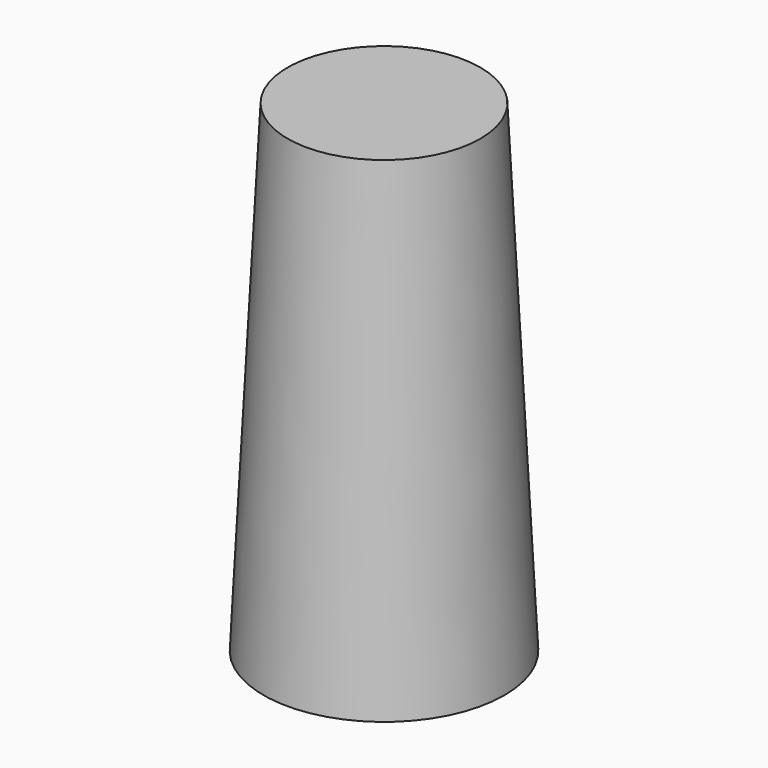
from build123d import *

# Parameters (mm, degrees)
F2_R = 6
F3_R = 7.5


with BuildPart() as f4:
    # F2 (on Top) → F4 section 0
    with BuildSketch(Plane.XY):
        Circle(F2_R)
    # F3 (on offset) → F4 section 1
    with BuildSketch(Plane.XY.offset(-30)):
        Circle(F3_R)
    loft()


solid = f4.part
